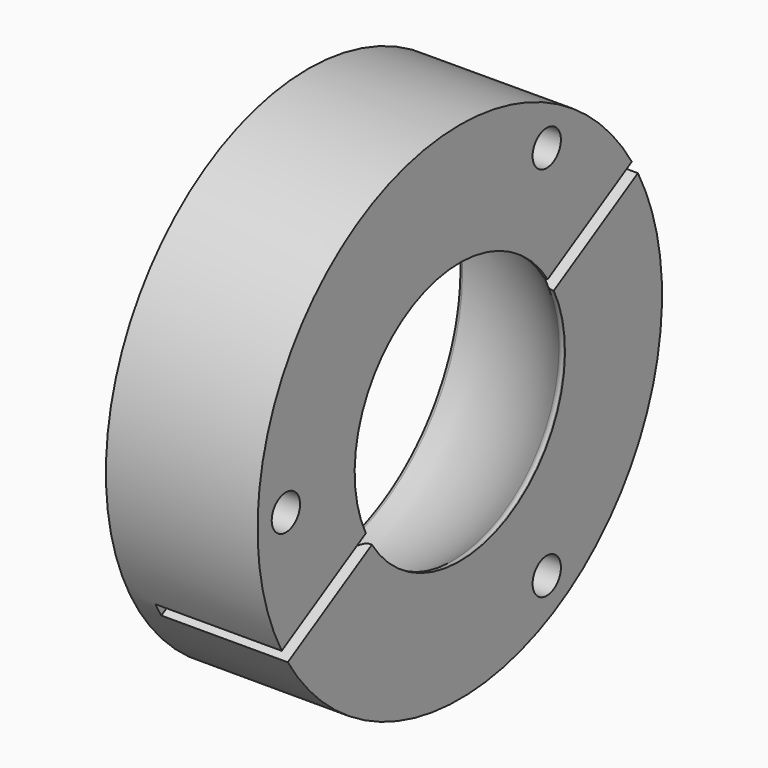
from build123d import *

# Parameters (mm, degrees)
F3_R            = 1
F4_R            = 3.5
F5_DEPTH        = 30.001
F5_COPIES_COUNT = 3
F7_DEPTH        = 25


# Not quite as in the source:
# - a fillet or chamfer that OpenCascade refuses, or shapes differently, is made with other operations: its cross-section is extruded or revolved along the edge and cut away or added
# - a pattern or mirror of a feature is missing from the dataset's text; its kind, count and spacing are read off the source's solid


with BuildPart() as f1:
    # F0 (on Front) → F1 (revolve)
    with BuildSketch(Plane.XZ):
        with BuildLine():
            Line((30, 50), (0, 50))
            Line((0, 50), (0, 37))
            ThreePointArc((0, 37), (15.5080624193, 34.1576191054), (29, 26))
            Line((29, 26), (30, 26))
            Line((30, 26), (30, 50))
        make_face()
    revolve(axis=Axis((-20.2939212322, 0, 0), (-1, 0, 0)))

    # F2: fillet of radius 2 on 1 edges, made by hand

    # F2_s1 → F2_t2 (revolve, cut)
    with BuildSketch(Plane.XZ):
        with BuildLine():
            ThreePointArc((29.7489495613, 26), (29.0553262341, 26.1241304203), (28.447802662, 26.4811133201))
            ThreePointArc((28.447802662, 26.4811133201), (28.7249086192, 26.241712774), (29, 26))
            Line((29, 26), (29.7489495613, 26))
        make_face()
    revolve(axis=Axis((29, 0, 0), (-1, 0, 0)), mode=Mode.SUBTRACT)

    # F3
    f3_edges = [f1.edges().sort_by_distance(p)[0] for p in [
        (0, 0, -37),
    ]]
    fillet(f3_edges, radius=F3_R)

    # F4 (on face) → F5 (cut, through all)
    with BuildSketch(Plane(origin=(0, 0, 0), x_dir=(0, -1, 0), z_dir=(-1, 0, 0))):
        with Locations((43, 0)):
            Circle(F4_R)
    f5 = extrude(amount=-F5_DEPTH, mode=Mode.SUBTRACT)

    # F5_copies: F5 ×3 about axis
    f5_copies_axis = Axis((0, 0, 0), (1, 0, 0))
    for i in range(1, F5_COPIES_COUNT):
        add(f5.rotate(f5_copies_axis, i * 360 / F5_COPIES_COUNT), mode=Mode.SUBTRACT)

    # F6 (on face) → F7 (cut)
    with BuildSketch(Plane.YZ.offset(30)):
        with BuildLine():
            ThreePointArc((44.0317802314, 23.6897093619), (43.3012701892, 25), (42.5317802314, 26.2877855733))
            Line((42.5317802314, 26.2877855733), (21.7291570127, 14.2773854581))
            ThreePointArc((21.7291570127, 14.2773854581), (22.5166604984, 13), (23.2291570127, 11.6793092467))
            Line((23.2291570127, 11.6793092467), (44.0317802314, 23.6897093619))
        make_face()
        with BuildLine():
            Line((-23.2291570127, -11.6793092467), (-44.0317802314, -23.6897093619))
            ThreePointArc((-44.0317802314, -23.6897093619), (-43.3012701892, -25), (-42.5317802314, -26.2877855733))
            Line((-42.5317802314, -26.2877855733), (-21.7291570127, -14.2773854581))
            ThreePointArc((-21.7291570127, -14.2773854581), (-22.5166604984, -13), (-23.2291570127, -11.6793092467))
        make_face()
    extrude(amount=-F7_DEPTH, mode=Mode.SUBTRACT)


solid = f1.part
